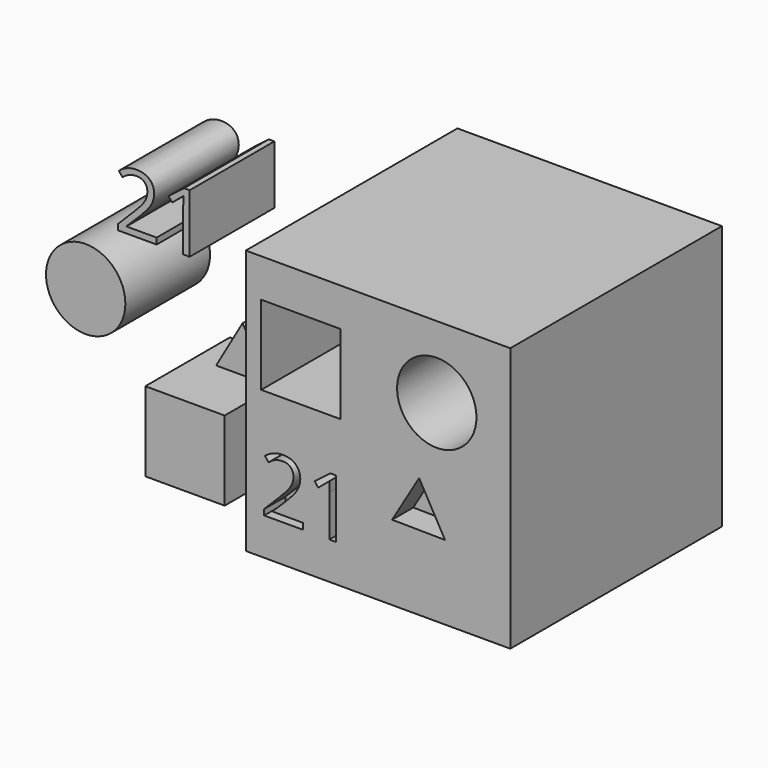
from build123d import *

# Parameters (mm, degrees)
F0_W          = 127
F0_H          = 127
F1_DEPTH      = 63.5
F2_W          = 38.1
F2_H          = 38.1
F3_DEPTH      = 50.8
F4_R          = 19.05
F5_DEPTH      = 38.1
F6_TEXT_SIZE  = 39.4161350818
F7_DEPTH      = 12.7
F9_DEPTH      = 12.7
F10_R         = 19.05
F11_DEPTH     = 50.8
F12_W         = 38.1
F12_H         = 38.1
F13_DEPTH     = 50.8
F14_TEXT_SIZE = 39.4161350818
F15_DEPTH     = 50.8
F17_DEPTH     = 25.4


# Not quite as in the source:
# - Text() gives the source's letters only with a copy of the font that has no kerning and outlines rounded to 1/6400 em; it was checked with that copy


with BuildPart() as f1:
    # F0 (on Front) → F1 (new body, symmetric)
    with BuildSketch(Plane.XZ):
        with Locations((11.983063072, 2.3737660095)):
            Rectangle(F0_W, F0_H)
    extrude(amount=F1_DEPTH, both=True)

    # F2 (on face) → F3 (cut)
    with BuildSketch(Plane.XZ.offset(63.5)):
        with Locations((-25.0591607764, 28.4480535567)):
            Rectangle(F2_W, F2_H)
    extrude(amount=-F3_DEPTH, mode=Mode.SUBTRACT)

    # F4 (on face) → F5 (cut)
    with BuildSketch(Plane.XZ.offset(63.5)):
        with Locations((40.1893556118, 31.3403233886)):
            Circle(F4_R)
    extrude(amount=-F5_DEPTH, mode=Mode.SUBTRACT)

    # F6 (on face) → F7 (cut, symmetric)
    with BuildSketch(Plane.XZ.offset(63.5)):
        with Locations((-44.5791347884, -43.2287408039)):
            Text('21', F6_TEXT_SIZE, font='Open Sans', text_align=(TextAlign.LEFT, TextAlign.BOTTOM))
    extrude(amount=F7_DEPTH, both=True, mode=Mode.SUBTRACT)

    # F8 (on face) → F9 (cut, symmetric)
    with BuildSketch(Plane.XZ.offset(63.5)):
        Polygon((18.746933789, -25.06741715), (44.1453380937, -25.3521253793), (31.6927005006, -3.2141079212), align=None)
    extrude(amount=F9_DEPTH, both=True, mode=Mode.SUBTRACT)


with BuildPart() as f11:
    # F10 (on Front) → F11 (new body)
    with BuildSketch(Plane.XZ):
        with Locations((-138.5349482064, 16.1239749573)):
            Circle(F10_R)
    extrude(amount=F11_DEPTH)


with BuildPart() as f13:
    # F12 (on Front) → F13 (new body)
    with BuildSketch(Plane.XZ):
        with Locations((-90.8647328615, -34.6852652729)):
            Rectangle(F12_W, F12_H)
    extrude(amount=F13_DEPTH)


with BuildPart() as f15:
    # F14 (on Front) → F15 (new body)
    with BuildSketch(Plane.XZ):
        with Locations((-124.8991787434, 45.9906831384)):
            Text('21', F14_TEXT_SIZE, font='Open Sans', text_align=(TextAlign.LEFT, TextAlign.BOTTOM))
    extrude(amount=F15_DEPTH)


with BuildPart() as f17:
    # F16 (on Front) → F17 (new body)
    with BuildSketch(Plane.XZ):
        Polygon((-83.535607424, 9.2551527673), (-96.235607424, -12.7418924888), (-70.835607424, -12.7418924888), align=None)
    extrude(amount=F17_DEPTH)


solid = Compound([f1.part, f11.part, f13.part, f15.part, f17.part])
